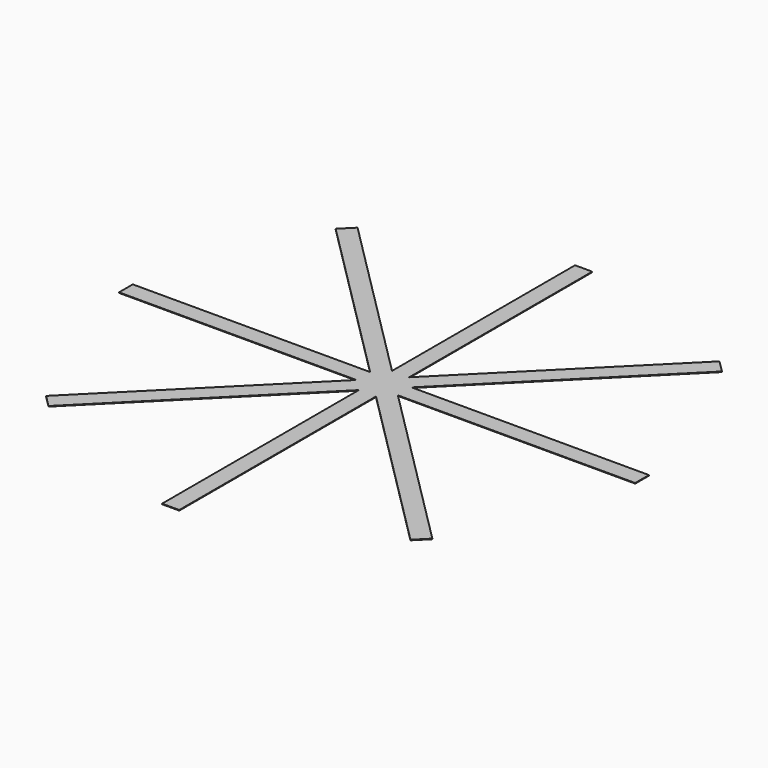
from build123d import *

# Parameters (mm, degrees)
F1_DEPTH = 0.2


# Not quite as in the source:
# - a feature names something its author has since deleted; it is built from what else it names


with BuildPart() as f1:
    # F0 (on Top) → F1 (new body)
    with BuildSketch(Plane.XY):
        Polygon((3, 87.0174653775), (-3, 87.0174653775), (-3, 7.2426406871), (-3, 3), (3, 3), (3, 7.2426406871), align=None)
        Polygon((-7.2426406871, 3), (-3, 7.2426406871), (-63.1040764009, 67.346717088), (-67.346717088, 63.1040764009), align=None)
        Polygon((-3, 3), (-3, 7.2426406871), (-7.2426406871, 3), align=None)
        Polygon((7.2426406871, 3), (3, 7.2426406871), (3, 3), align=None)
        Polygon((63.1040764009, 67.346717088), (3, 7.2426406871), (7.2426406871, 3), (67.346717088, 63.1040764009), align=None)
        Polygon((3, 3), (-3, 3), (-3, 0), (0, 0), (3, 0), align=None)
        Polygon((-3, 0), (-3, 3), (-7.2426406871, 3), (-90, 3), (-90, -3), (-7.2426406871, -3), (-3, -3), align=None)
        Polygon((7.2426406871, 3), (3, 3), (3, 0), (3, -3), (7.2426406871, -3), (90, -3), (90, 3), align=None)
        Polygon((0, 0), (-3, 0), (-3, -3), (3, -3), (3, 0), align=None)
        Polygon((3, -3), (-3, -3), (-3, -7.2426406871), (-3, -92.9825346225), (3, -92.9825346225), (3, -7.2426406871), align=None)
        Polygon((-3, -7.2426406871), (-3, -3), (-7.2426406871, -3), align=None)
        Polygon((7.2426406871, -3), (3, -3), (3, -7.2426406871), align=None)
        Polygon((-63.1040764009, -67.346717088), (-3, -7.2426406871), (-7.2426406871, -3), (-67.346717088, -63.1040764009), align=None)
        Polygon((7.2426406871, -3), (3, -7.2426406871), (63.1040764009, -67.346717088), (67.346717088, -63.1040764009), align=None)
    extrude(amount=F1_DEPTH)


solid = f1.part
